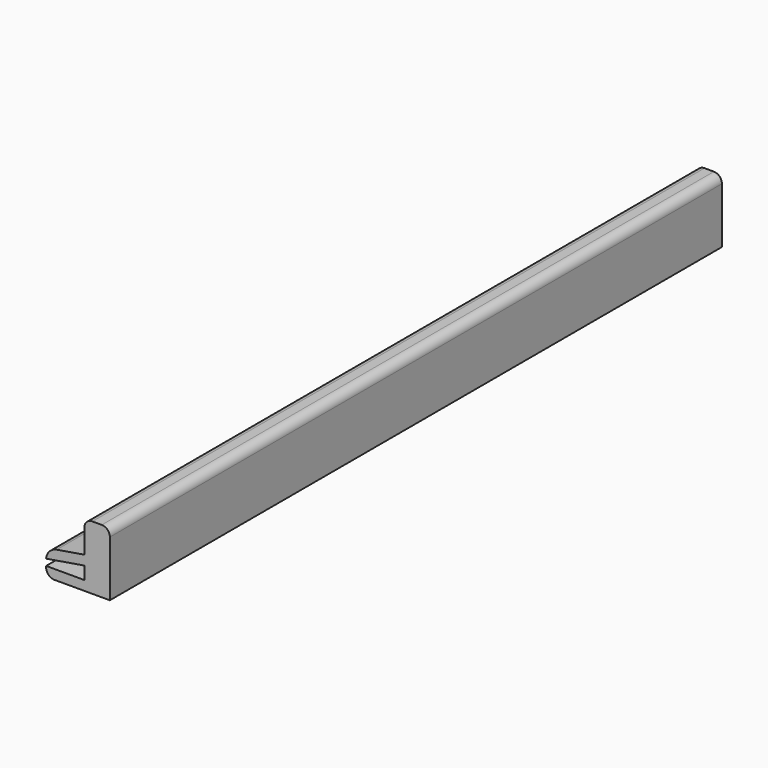
from build123d import *

# Parameters (mm, degrees)
F0_W        = 9
F0_H        = 2.25
F1_DEPTH    = 180
F2_T1_DEPTH = 192.6338141032
F3_R        = 2
F4_R        = 1.9


# Not quite as in the source:
# - a fillet or chamfer that OpenCascade refuses, or shapes differently, is made with other operations: its cross-section is extruded or revolved along the edge and cut away or added


with BuildPart() as f1:
    # F0 (on Front) → F1 (new body)
    with BuildSketch(Plane.XZ):
        Polygon((1.5, -2.25), (1.5, 0), (-7.5, -1.5), (-7.5, -3.75), align=None)
        Polygon((7.5, -7.5), (7.5, 7.5), (1.5, 7.5), (1.5, 0), (1.5, -2.25), (1.5, -5.25), (1.5, -7.5), align=None)
        with Locations((-3, -6.375)):
            Rectangle(F0_W, F0_H)
    extrude(amount=-F1_DEPTH)

    # F2: fillet of radius 3 on 1 edges, made by hand

    # F2_s2 → F2_t1 (cut)
    with BuildSketch(Plane.XZ.offset(-186.3169070516)):
        with BuildLine():
            ThreePointArc((-5.0076165068, -1.0846027511), (-6.7056654696, -1.9947746893), (-7.5, -3.75))
            Line((-7.5, -3.75), (-7.5, -1.5))
            Line((-7.5, -1.5), (-5.0076165068, -1.0846027511))
        make_face()
    extrude(amount=F2_T1_DEPTH, mode=Mode.SUBTRACT)

    # F3
    f3_edges = [f1.edges().sort_by_distance(p)[0] for p in [
        (-7.5, 90, -7.5),
    ]]
    fillet(f3_edges, radius=F3_R)

    # F4
    f4_edges = [f1.edges().sort_by_distance(p)[0] for p in [
        (1.5, 90, 7.5),
        (7.5, 90, 7.5),
    ]]
    fillet(f4_edges, radius=F4_R)


solid = f1.part
